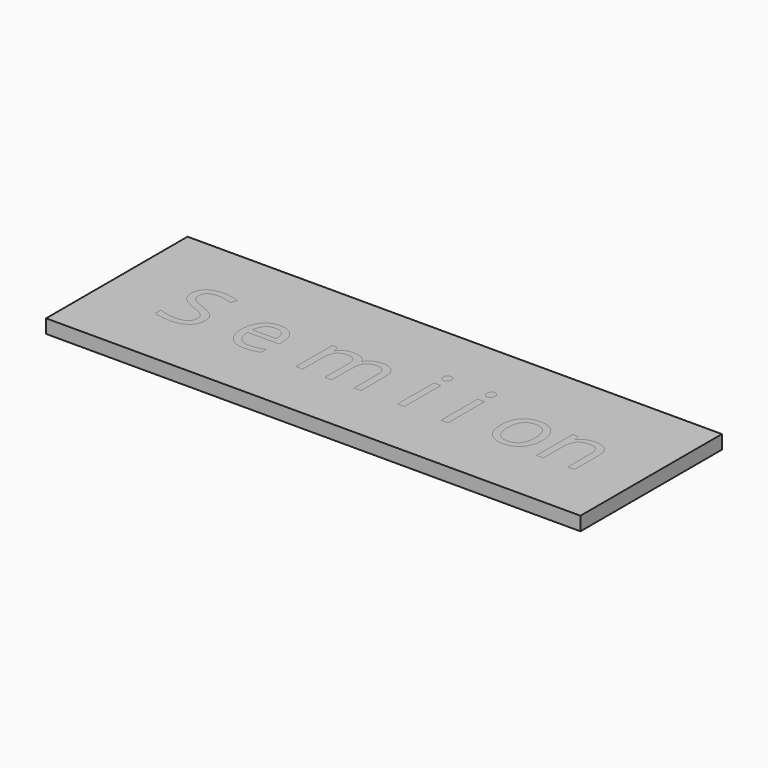
from build123d import *

# Parameters (mm, degrees)
F1_W         = 116.602233611
F1_H         = 38.5862728581
F2_DEPTH     = 3
F0_TEXT_SIZE = 18.6215736903
F3_DEPTH     = 2
F4_DEPTH     = 2


# Not quite as in the source:
# - Text() gives the source's letters only with a copy of the font that has no kerning and outlines rounded to 1/6400 em; it was checked with that copy


with BuildPart() as f2:
    # F1 (on Top) → F2 (new body)
    with BuildSketch(Plane.XY):
        with Locations((-48.0828699656, 6.6046942957)):
            Rectangle(F1_W, F1_H)
    extrude(amount=-F2_DEPTH)

    # F0 (on Top) → F3 (cut)
    with BuildSketch(Plane.XY):
        with Locations((-93.9923932019, 0)):
            Text('S e m i i on', F0_TEXT_SIZE, font='Open Sans', text_align=(TextAlign.LEFT, TextAlign.BOTTOM))
    extrude(amount=-F3_DEPTH, mode=Mode.SUBTRACT)


with BuildPart() as f4:
    # F0 (on Top) → F4 (new body)
    with BuildSketch(Plane.XY):
        with Locations((-93.9923932019, 0)):
            Text('S e m i i on', F0_TEXT_SIZE, font='Open Sans', text_align=(TextAlign.LEFT, TextAlign.BOTTOM))
    extrude(amount=-F4_DEPTH)


solid = Compound([f2.part, f4.part])
